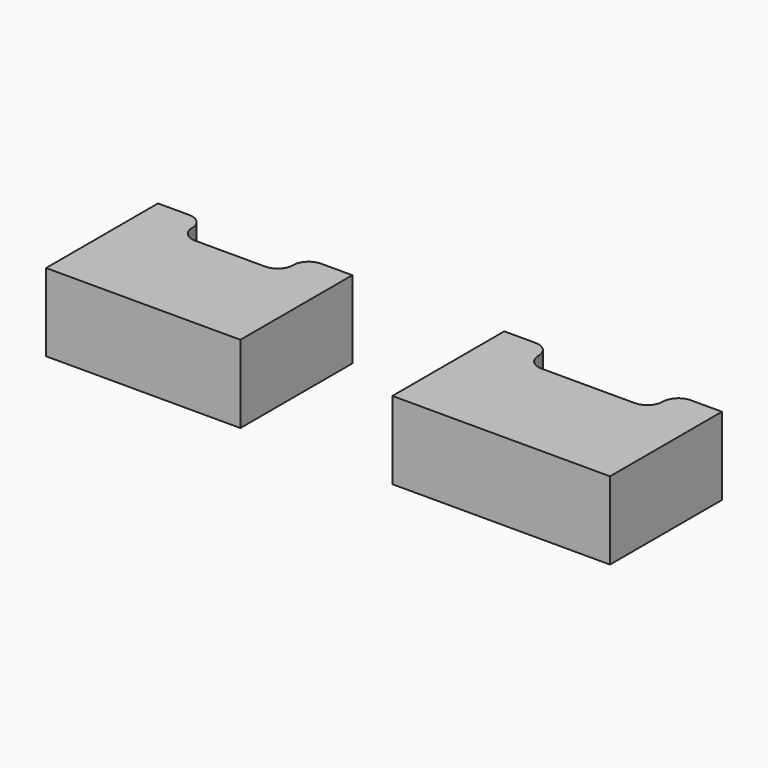
from build123d import *

# Parameters (mm, degrees)
F0_W     = 25
F0_H     = 18
F1_DEPTH = 10
F2_W     = 13
F2_H     = 4
F3_DEPTH = 10.001
F4_W     = 28
F4_H     = 18
F5_DEPTH = 10
F6_W     = 16
F6_H     = 4
F7_DEPTH = 10.001
F8_R     = 1.99999
F8_2_R   = 1.99999


# Not quite as in the source:
# - a fillet or chamfer is up to 0.001 mm smaller than in the source, because OpenCascade refuses the exact size


with BuildPart() as f1:
    # F0 (on Top) → F1 (new body)
    with BuildSketch(Plane.XY):
        with Locations((12.5, 9)):
            Rectangle(F0_W, F0_H)
    extrude(amount=F1_DEPTH)

    # F2 (on Top) → F3 (cut, through all)
    with BuildSketch(Plane.XY):
        with Locations((12.5, 16)):
            Rectangle(F2_W, F2_H)
    extrude(amount=F3_DEPTH, mode=Mode.SUBTRACT)

    # F8 (radius 2 in the source; OpenCascade refuses exactly that, so slightly less here)
    f8_edges = [f1.edges().sort_by_distance(p)[0] for p in [
        (6, 14, 5),
        (19, 14, 5),
        (6, 18, 5),
        (19, 18, 5),
    ]]
    fillet(f8_edges, radius=F8_R)


with BuildPart() as f5:
    # F4 (on Top) → F5 (new body)
    with BuildSketch(Plane.XY):
        with Locations((58.5543287322, 9)):
            Rectangle(F4_W, F4_H)
    extrude(amount=F5_DEPTH)

    # F6 (on Top) → F7 (cut, through all)
    with BuildSketch(Plane.XY):
        with Locations((58.5543287322, 16)):
            Rectangle(F6_W, F6_H)
    extrude(amount=F7_DEPTH, mode=Mode.SUBTRACT)

    # F8#2 (radius 2 in the source; OpenCascade refuses exactly that, so slightly less here)
    f8_2_edges = [f5.edges().sort_by_distance(p)[0] for p in [
        (50.554329, 18, 5),
        (50.554329, 14, 5),
        (66.554329, 14, 5),
        (66.554329, 18, 5),
    ]]
    fillet(f8_2_edges, radius=F8_2_R)


solid = Compound([f1.part, f5.part])
